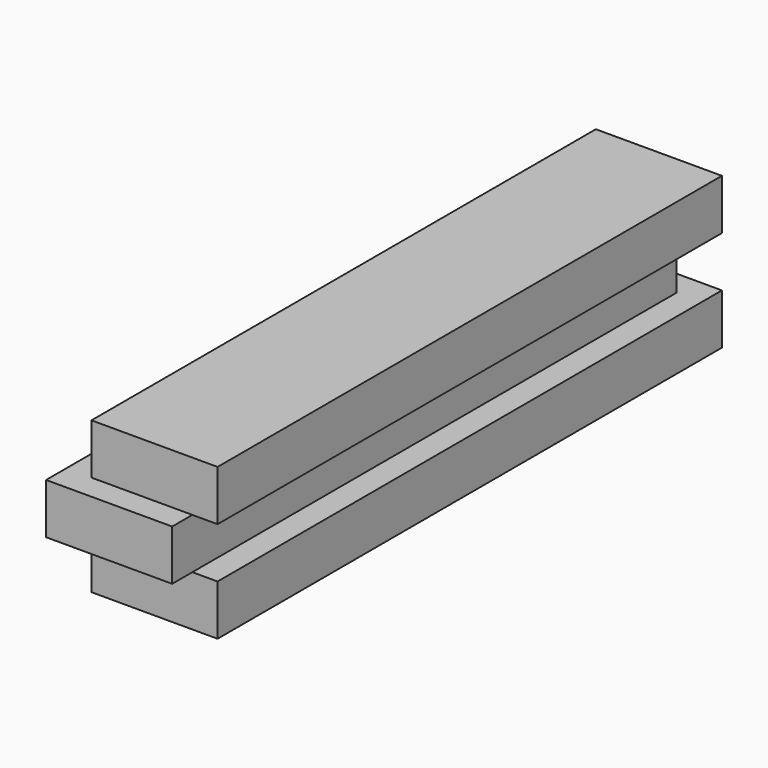
from build123d import *

# Parameters (mm, degrees)
F2_W     = 7.9375
F2_H     = 39.6875
F3_DEPTH = 3.175
F4_W     = 7.9375
F4_H     = 39.6875
F5_DEPTH = 3.175
F6_W     = 7.9375
F6_H     = 39.6875
F7_DEPTH = 3.175


# Not quite as in the source:
# - a variable given as a bare number and used for a length is read in inches; the dataset says mm whatever the document's units were


with BuildPart() as f3:
    # F2 (on Top) → F3 (new body)
    with BuildSketch(Plane.XY):
        with Locations((3.96875, 19.84375)):
            Rectangle(F2_W, F2_H)
    extrude(amount=F3_DEPTH)

    # F4 (on face) → F5 (join)
    with BuildSketch(Plane.XY.offset(3.175)):
        with Locations((2.38125, 18.25625)):
            Rectangle(F4_W, F4_H)
    extrude(amount=F5_DEPTH)

    # F6 (on face) → F7 (join)
    with BuildSketch(Plane.XY.offset(6.35)):
        with Locations((3.96875, 19.84375)):
            Rectangle(F6_W, F6_H)
    extrude(amount=F7_DEPTH)


solid = f3.part
